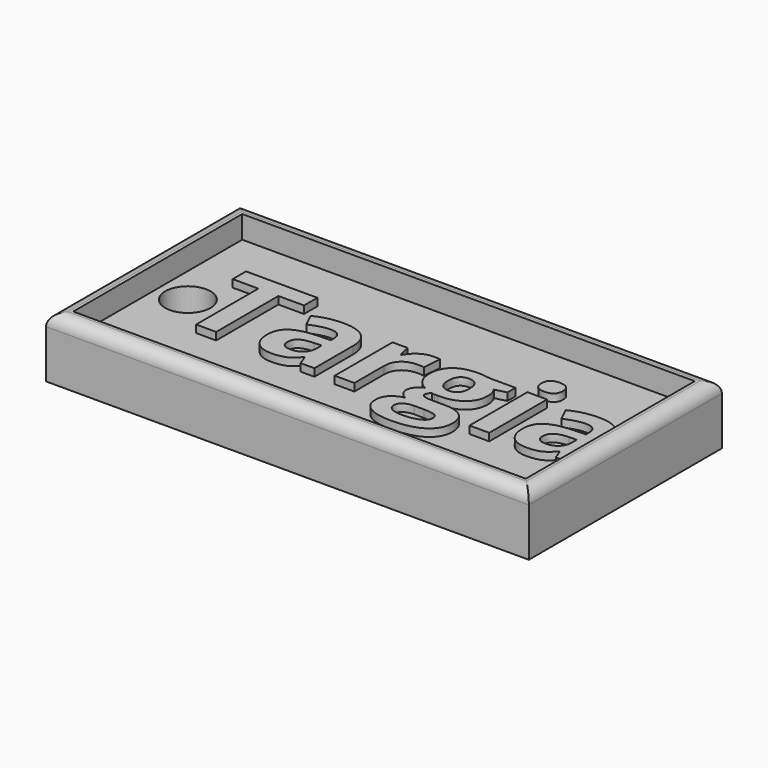
from build123d import *

# Parameters (mm, degrees)
F0_W         = 47.625
F0_H         = 22.225
F0_R         = 2.38125
F1_DEPTH     = 4.7625
F0_W_2       = 50.8
F0_H_2       = 25.4
F2_DEPTH     = 6.35
F3_R         = 1.27
F4_DEPTH     = 1.5875
F5_DEPTH     = 0.79375
F6_TEXT_SIZE = 13.9248211226
F7_DEPTH     = 0.79375


# Not quite as in the source:
# - Text() gives the source's letters only with a copy of the font that has no kerning and outlines rounded to 1/6400 em; it was checked with that copy


with BuildPart() as f1:
    # F0 (on Top) → F1 (new body)
    with BuildSketch(Plane.XY):
        with Locations((25.4, 12.7)):
            Rectangle(F0_W, F0_H)
        with Locations((4.7625, 12.7)):
            Circle(F0_R, mode=Mode.SUBTRACT)
    extrude(amount=F1_DEPTH)

    # F0 (on Top) → F2 (join)
    with BuildSketch(Plane.XY):
        with Locations((25.4, 12.7)):
            Rectangle(F0_W_2, F0_H_2)
        with Locations((25.4, 12.7)):
            Rectangle(F0_W, F0_H, mode=Mode.SUBTRACT)
    extrude(amount=F2_DEPTH)

    # F3
    f3_edges = [f1.edges().sort_by_distance(p)[0] for p in [
        (25.4, 0, 6.35),
        (50.8, 12.7, 6.35),
        (25.4, 25.4, 6.35),
        (0, 12.7, 6.35),
    ]]
    fillet(f3_edges, radius=F3_R)

    # F4 (cut): a face of the model
    f4_faces = [f1.faces().sort_by_distance(p)[0] for p in [
        (25.7532738986, 12.7, 4.7625),
    ]]
    extrude(f4_faces, amount=-F4_DEPTH, mode=Mode.SUBTRACT)

    # F5 (add): a face of the model
    f5_faces = [f1.faces().sort_by_distance(p)[0] for p in [
        (25.7532738986, 12.7, 3.175),
    ]]
    extrude(f5_faces, amount=F5_DEPTH)

    # F6 (on face) → F7 (join)
    with BuildSketch(Plane.XY.offset(3.96875)):
        with Locations((6.0325, 8.4706579318)):
            Text('Targia', F6_TEXT_SIZE, font='Open Sans', font_style=FontStyle.BOLD, text_align=(TextAlign.LEFT, TextAlign.BOTTOM))
    extrude(amount=F7_DEPTH)


solid = f1.part
